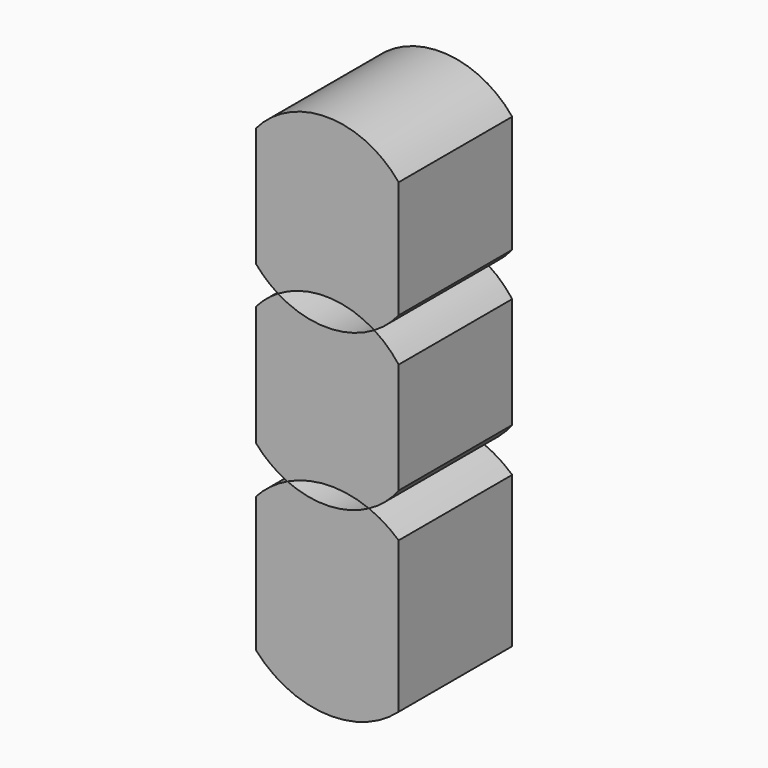
from build123d import *

# Parameters (mm, degrees)
F1_DEPTH = 25.4


with BuildPart() as f1:
    # F0 (on Front) → F1 (new body)
    with BuildSketch(Plane.XZ):
        with BuildLine():
            ThreePointArc((2.9849638231, 55.841046589), (-9.7614743803, 61.9401882116), (-22.581897676, 55.9981378983))
            Line((-22.581897676, 55.9981378983), (-22.581897676, 34.7187977959))
            ThreePointArc((-22.581897676, 34.7187977959), (-20.7339157895, 32.8366946633), (-18.6108785729, 31.2714272002))
            ThreePointArc((-18.6108785729, 31.2714272002), (-9.9714363538, 33.6319387195), (-1.3769697054, 31.1125896929))
            ThreePointArc((-1.3769697054, 31.1125896929), (0.9686810311, 32.8033588814), (2.9849638231, 34.8758891053))
            Line((2.9849638231, 34.8758891053), (2.9849638231, 55.841046589))
        make_face()
    extrude(amount=F1_DEPTH)


with BuildPart() as f1b:
    # F0 (on Front) → F1, piece 2 (new body)
    with BuildSketch(Plane.XZ):
        with BuildLine():
            ThreePointArc((-18.6108785729, 31.2714272002), (-20.7298421272, 29.7521275364), (-22.581897676, 27.9168705362))
            Line((-22.581897676, 27.9168705362), (-22.581897676, 6.4750989062))
            ThreePointArc((-22.581897676, 6.4750989062), (-19.9904965776, 4.0508543415), (-16.9391677392, 2.2393042641))
            ThreePointArc((-16.9391677392, 2.2393042641), (-9.6855767528, 4.0210300271), (-2.3297951619, 2.7242624769))
            ThreePointArc((-2.3297951619, 2.7242624769), (0.5728460014, 4.7154345625), (2.9849638231, 7.2789828089))
            Line((2.9849638231, 7.2789828089), (2.9849638231, 27.1129866335))
            ThreePointArc((2.9849638231, 27.1129866335), (0.9854877512, 29.3107203891), (-1.3769697054, 31.1125896929))
            ThreePointArc((-1.3769697054, 31.1125896929), (-10.0161809522, 28.7771387188), (-18.6108785729, 31.2714272002))
        make_face()
    extrude(amount=F1_DEPTH)


with BuildPart() as f1c:
    # F0 (on Front) → F1, piece 3 (new body)
    with BuildSketch(Plane.XZ):
        with BuildLine():
            ThreePointArc((-16.9391677392, 2.2393042641), (-19.9692385493, 0.3956202808), (-22.581897676, -2.00323612))
            Line((-22.581897676, -2.00323612), (-22.581897676, -26.1592470059))
            ThreePointArc((-22.581897676, -26.1592470059), (-10.0938178152, -32.1653491647), (2.9849638231, -27.5859526312))
            Line((2.9849638231, -27.5859526312), (2.9849638231, -0.5765304947))
            ThreePointArc((2.9849638231, -0.5765304947), (0.4711836848, 1.3050819337), (-2.3297951619, 2.7242624769))
            ThreePointArc((-2.3297951619, 2.7242624769), (-9.5776050492, 0.7683810261), (-16.9391677392, 2.2393042641))
        make_face()
    extrude(amount=F1_DEPTH)


solid = Compound([f1.part, f1b.part, f1c.part])
